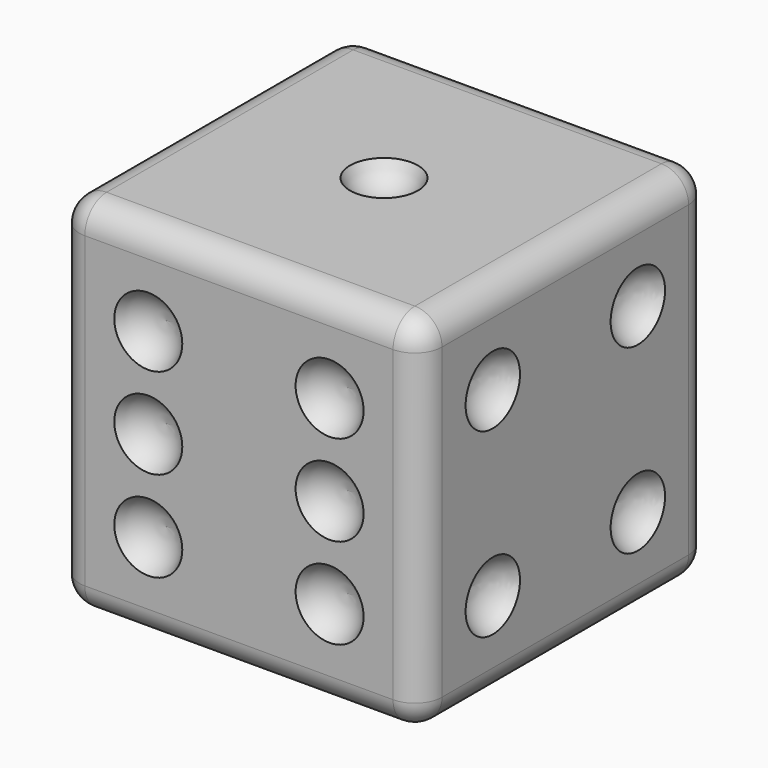
from build123d import *

# Parameters (mm, degrees)
F0_W      = 101.6
F0_H      = 101.6
F0_R      = 9.525
F1_DEPTH  = 101.6
F2_R      = 9.525
F3_DEPTH  = 6.35
F5_R      = 9.525
F6_DEPTH  = 6.35
F8_R      = 9.525
F9_DEPTH  = 6.35
F11_R     = 9.525
F12_DEPTH = 6.35
F14_R     = 9.525
F15_DEPTH = 6.35
F17_R     = 9.525
F18_DEPTH = 6.35
F20_R     = 7.62


# Not quite as in the source:
# - a fillet or chamfer that OpenCascade refuses, or shapes differently, is made with other operations: its cross-section is extruded or revolved along the edge and cut away or added


with BuildPart() as f1:
    # F0 (on Top) → F1 (new body)
    with BuildSketch(Plane.XY):
        with Locations((4.8996444777, 3.5687691152)):
            Rectangle(F0_W, F0_H)
        with Locations((4.8996444777, 3.5687691152)):
            Circle(F0_R, mode=Mode.SUBTRACT)
        with Locations((4.8996444777, 3.5687691152)):
            Circle(F0_R)
    extrude(amount=F1_DEPTH)

    # F2 (on face) → F3 (cut)
    with BuildSketch(Plane.XY.offset(101.6)):
        with Locations((4.8996444777, 3.5687691152)):
            Circle(F2_R)
    extrude(amount=-F3_DEPTH, mode=Mode.SUBTRACT)

    # F4: fillet of radius 10.16 on 1 edges, made by hand

    # F4_s1 → F4_t2 (revolve)
    with BuildSketch(Plane.XZ.offset(-3.5687691152)):
        with BuildLine():
            ThreePointArc((14.4246444777, 101.6), (10.685685062, 96.9857730325), (5.0060723991, 95.25))
            Line((5.0060723991, 95.25), (14.4246444777, 95.25))
            Line((14.4246444777, 95.25), (14.4246444777, 101.6))
        make_face()
    revolve(axis=Axis((4.8996444777, 3.5687691152, 95.25), (0, 0, 1)))

    # F5 (on face) → F6 (cut)
    with BuildSketch(Plane(origin=(-45.9003555223, 0, 0), x_dir=(0, -1, 0), z_dir=(-1, 0, 0))):
        with Locations((-28.9687691152, 25.4)):
            Circle(F5_R)
        with Locations((21.8312308848, 76.2)):
            Circle(F5_R)
    extrude(amount=-F6_DEPTH, mode=Mode.SUBTRACT)

    # F7: fillet of radius 10.16 on 2 edges, made by hand

    # F7_s1 → F7_t2 (revolve)
    with BuildSketch(Plane.XY.offset(25.4)):
        with BuildLine():
            ThreePointArc((-45.9003555223, 19.4437691152), (-41.2861285547, 23.182728531), (-39.5503555223, 28.8623411938))
            Line((-39.5503555223, 28.8623411938), (-39.5503555223, 19.4437691152))
            Line((-39.5503555223, 19.4437691152), (-45.9003555223, 19.4437691152))
        make_face()
    revolve(axis=Axis((-39.5503555223, 28.9687691152, 25.4), (-1, 0, 0)))

    # F7_s3 → F7_t4 (revolve)
    with BuildSketch(Plane.XY.offset(76.2)):
        with BuildLine():
            ThreePointArc((-45.9003555223, -31.3562308848), (-41.2861285547, -27.617271469), (-39.5503555223, -21.9376588062))
            Line((-39.5503555223, -21.9376588062), (-39.5503555223, -31.3562308848))
            Line((-39.5503555223, -31.3562308848), (-45.9003555223, -31.3562308848))
        make_face()
    revolve(axis=Axis((-39.5503555223, -21.8312308848, 76.2), (-1, 0, 0)))

    # F8 (on face) → F9 (cut)
    with BuildSketch(Plane(origin=(0, 0, 0), x_dir=(1, 0, 0), z_dir=(0, 0, -1))):
        with Locations((4.8996444777, -3.5687691152)):
            Circle(F8_R)
        with Locations((30.2996444777, 21.8312308848)):
            Circle(F8_R)
        with Locations((-20.5003555223, -28.9687691152)):
            Circle(F8_R)
    extrude(amount=-F9_DEPTH, mode=Mode.SUBTRACT)

    # F10: fillet of radius 10.16 on 3 edges, made by hand

    # F10_s1 → F10_t2 (revolve)
    with BuildSketch(Plane.XZ.offset(-28.9687691152)):
        with BuildLine():
            ThreePointArc((-10.9753555223, 0), (-14.714314938, 4.6142269675), (-20.3939276009, 6.35))
            Line((-20.3939276009, 6.35), (-10.9753555223, 6.35))
            Line((-10.9753555223, 6.35), (-10.9753555223, 0))
        make_face()
    revolve(axis=Axis((-20.5003555223, 28.9687691152, 6.35), (0, 0, -1)))

    # F10_s3 → F10_t4 (revolve)
    with BuildSketch(Plane.XZ.offset(-3.5687691152)):
        with BuildLine():
            ThreePointArc((14.4246444777, 0), (10.685685062, 4.6142269675), (5.0060723991, 6.35))
            Line((5.0060723991, 6.35), (14.4246444777, 6.35))
            Line((14.4246444777, 6.35), (14.4246444777, 0))
        make_face()
    revolve(axis=Axis((4.8996444777, 3.5687691152, 6.35), (0, 0, -1)))

    # F10_s5 → F10_t6 (revolve)
    with BuildSketch(Plane.XZ.offset(21.8312308848)):
        with BuildLine():
            ThreePointArc((39.8246444777, 0), (36.085685062, 4.6142269675), (30.4060723991, 6.35))
            Line((30.4060723991, 6.35), (39.8246444777, 6.35))
            Line((39.8246444777, 6.35), (39.8246444777, 0))
        make_face()
    revolve(axis=Axis((30.2996444777, -21.8312308848, 6.35), (0, 0, -1)))

    # F11 (on face) → F12 (cut)
    with BuildSketch(Plane.YZ.offset(55.6996444777)):
        with Locations((-21.8312308848, 25.4)):
            Circle(F11_R)
        with Locations((-21.8312308848, 76.2)):
            Circle(F11_R)
        with Locations((28.9687691152, 25.4)):
            Circle(F11_R)
        with Locations((28.9687691152, 76.2)):
            Circle(F11_R)
    extrude(amount=-F12_DEPTH, mode=Mode.SUBTRACT)

    # F13: fillet of radius 10.16 on 4 edges, made by hand

    # F13_s1 → F13_t2 (revolve)
    with BuildSketch(Plane.XY.offset(25.4)):
        with BuildLine():
            ThreePointArc((55.6996444777, 38.4937691152), (51.0854175102, 34.7548096994), (49.3496444777, 29.0751970366))
            Line((49.3496444777, 29.0751970366), (49.3496444777, 38.4937691152))
            Line((49.3496444777, 38.4937691152), (55.6996444777, 38.4937691152))
        make_face()
    revolve(axis=Axis((49.3496444777, 28.9687691152, 25.4), (1, 0, 0)))

    # F13_s3 → F13_t4 (revolve)
    with BuildSketch(Plane.XY.offset(76.2)):
        with BuildLine():
            ThreePointArc((55.6996444777, 38.4937691152), (51.0854175102, 34.7548096994), (49.3496444777, 29.0751970366))
            Line((49.3496444777, 29.0751970366), (49.3496444777, 38.4937691152))
            Line((49.3496444777, 38.4937691152), (55.6996444777, 38.4937691152))
        make_face()
    revolve(axis=Axis((49.3496444777, 28.9687691152, 76.2), (1, 0, 0)))

    # F13_s5 → F13_t6 (revolve)
    with BuildSketch(Plane.XY.offset(76.2)):
        with BuildLine():
            ThreePointArc((55.6996444777, -12.3062308848), (51.0854175102, -16.0451903006), (49.3496444777, -21.7248029634))
            Line((49.3496444777, -21.7248029634), (49.3496444777, -12.3062308848))
            Line((49.3496444777, -12.3062308848), (55.6996444777, -12.3062308848))
        make_face()
    revolve(axis=Axis((49.3496444777, -21.8312308848, 76.2), (1, 0, 0)))

    # F13_s7 → F13_t8 (revolve)
    with BuildSketch(Plane.XY.offset(25.4)):
        with BuildLine():
            ThreePointArc((55.6996444777, -12.3062308848), (51.0854175102, -16.0451903006), (49.3496444777, -21.7248029634))
            Line((49.3496444777, -21.7248029634), (49.3496444777, -12.3062308848))
            Line((49.3496444777, -12.3062308848), (55.6996444777, -12.3062308848))
        make_face()
    revolve(axis=Axis((49.3496444777, -21.8312308848, 25.4), (1, 0, 0)))

    # F14 (on face) → F15 (cut)
    with BuildSketch(Plane(origin=(0, 54.3687691152, 0), x_dir=(-1, 0, 0), z_dir=(0, 1, 0))):
        with Locations((-4.8996444777, 50.8)):
            Circle(F14_R)
        with Locations((-30.2996444777, 25.4)):
            Circle(F14_R)
        with Locations((20.5003555223, 76.2)):
            Circle(F14_R)
        with Locations((-30.2996444777, 76.2)):
            Circle(F14_R)
        with Locations((20.5003555223, 25.4)):
            Circle(F14_R)
    extrude(amount=-F15_DEPTH, mode=Mode.SUBTRACT)

    # F16: fillet of radius 10.16 on 5 edges, made by hand

    # F16_s1 → F16_t2 (revolve)
    with BuildSketch(Plane.XY.offset(25.4)):
        with BuildLine():
            ThreePointArc((-30.0253555223, 54.3687691152), (-26.2863961065, 49.7545421477), (-20.6067834436, 48.0187691152))
            Line((-20.6067834436, 48.0187691152), (-30.0253555223, 48.0187691152))
            Line((-30.0253555223, 48.0187691152), (-30.0253555223, 54.3687691152))
        make_face()
    revolve(axis=Axis((-20.5003555223, 48.0187691152, 25.4), (0, 1, 0)))

    # F16_s3 → F16_t4 (revolve)
    with BuildSketch(Plane.XY.offset(50.8)):
        with BuildLine():
            ThreePointArc((-4.6253555223, 54.3687691152), (-0.8863961065, 49.7545421477), (4.7932165564, 48.0187691152))
            Line((4.7932165564, 48.0187691152), (-4.6253555223, 48.0187691152))
            Line((-4.6253555223, 48.0187691152), (-4.6253555223, 54.3687691152))
        make_face()
    revolve(axis=Axis((4.8996444777, 48.0187691152, 50.8), (0, 1, 0)))

    # F16_s5 → F16_t6 (revolve)
    with BuildSketch(Plane.XY.offset(76.2)):
        with BuildLine():
            ThreePointArc((-30.0253555223, 54.3687691152), (-26.2863961065, 49.7545421477), (-20.6067834436, 48.0187691152))
            Line((-20.6067834436, 48.0187691152), (-30.0253555223, 48.0187691152))
            Line((-30.0253555223, 48.0187691152), (-30.0253555223, 54.3687691152))
        make_face()
    revolve(axis=Axis((-20.5003555223, 48.0187691152, 76.2), (0, 1, 0)))

    # F16_s7 → F16_t8 (revolve)
    with BuildSketch(Plane.XY.offset(76.2)):
        with BuildLine():
            ThreePointArc((20.7746444777, 54.3687691152), (24.5136038935, 49.7545421477), (30.1932165564, 48.0187691152))
            Line((30.1932165564, 48.0187691152), (20.7746444777, 48.0187691152))
            Line((20.7746444777, 48.0187691152), (20.7746444777, 54.3687691152))
        make_face()
    revolve(axis=Axis((30.2996444777, 48.0187691152, 76.2), (0, 1, 0)))

    # F16_s9 → F16_t10 (revolve)
    with BuildSketch(Plane.XY.offset(25.4)):
        with BuildLine():
            ThreePointArc((20.7746444777, 54.3687691152), (24.5136038935, 49.7545421477), (30.1932165564, 48.0187691152))
            Line((30.1932165564, 48.0187691152), (20.7746444777, 48.0187691152))
            Line((20.7746444777, 48.0187691152), (20.7746444777, 54.3687691152))
        make_face()
    revolve(axis=Axis((30.2996444777, 48.0187691152, 25.4), (0, 1, 0)))

    # F17 (on face) → F18 (cut)
    with BuildSketch(Plane.XZ.offset(47.2312308848)):
        with Locations((30.2996444777, 25.4)):
            Circle(F17_R)
        with Locations((30.2996444777, 50.8)):
            Circle(F17_R)
        with Locations((30.2996444777, 76.2)):
            Circle(F17_R)
        with Locations((-20.5003555223, 25.4)):
            Circle(F17_R)
        with Locations((-20.5003555223, 50.8)):
            Circle(F17_R)
        with Locations((-20.5003555223, 76.2)):
            Circle(F17_R)
    extrude(amount=-F18_DEPTH, mode=Mode.SUBTRACT)

    # F19: fillet of radius 10.16 on 6 edges, made by hand

    # F19_s1 → F19_t2 (revolve)
    with BuildSketch(Plane.XY.offset(25.4)):
        with BuildLine():
            ThreePointArc((39.8246444777, -47.2312308848), (36.085685062, -42.6170039173), (30.4060723991, -40.8812308848))
            Line((30.4060723991, -40.8812308848), (39.8246444777, -40.8812308848))
            Line((39.8246444777, -40.8812308848), (39.8246444777, -47.2312308848))
        make_face()
    revolve(axis=Axis((30.2996444777, -40.8812308848, 25.4), (0, -1, 0)))

    # F19_s3 → F19_t4 (revolve)
    with BuildSketch(Plane.XY.offset(50.8)):
        with BuildLine():
            ThreePointArc((39.8246444777, -47.2312308848), (36.085685062, -42.6170039173), (30.4060723991, -40.8812308848))
            Line((30.4060723991, -40.8812308848), (39.8246444777, -40.8812308848))
            Line((39.8246444777, -40.8812308848), (39.8246444777, -47.2312308848))
        make_face()
    revolve(axis=Axis((30.2996444777, -40.8812308848, 50.8), (0, -1, 0)))

    # F19_s5 → F19_t6 (revolve)
    with BuildSketch(Plane.XY.offset(76.2)):
        with BuildLine():
            ThreePointArc((39.8246444777, -47.2312308848), (36.085685062, -42.6170039173), (30.4060723991, -40.8812308848))
            Line((30.4060723991, -40.8812308848), (39.8246444777, -40.8812308848))
            Line((39.8246444777, -40.8812308848), (39.8246444777, -47.2312308848))
        make_face()
    revolve(axis=Axis((30.2996444777, -40.8812308848, 76.2), (0, -1, 0)))

    # F19_s7 → F19_t8 (revolve)
    with BuildSketch(Plane.XY.offset(76.2)):
        with BuildLine():
            ThreePointArc((-10.9753555223, -47.2312308848), (-14.714314938, -42.6170039173), (-20.3939276009, -40.8812308848))
            Line((-20.3939276009, -40.8812308848), (-10.9753555223, -40.8812308848))
            Line((-10.9753555223, -40.8812308848), (-10.9753555223, -47.2312308848))
        make_face()
    revolve(axis=Axis((-20.5003555223, -40.8812308848, 76.2), (0, -1, 0)))

    # F19_s9 → F19_t10 (revolve)
    with BuildSketch(Plane.XY.offset(50.8)):
        with BuildLine():
            ThreePointArc((-10.9753555223, -47.2312308848), (-14.714314938, -42.6170039173), (-20.3939276009, -40.8812308848))
            Line((-20.3939276009, -40.8812308848), (-10.9753555223, -40.8812308848))
            Line((-10.9753555223, -40.8812308848), (-10.9753555223, -47.2312308848))
        make_face()
    revolve(axis=Axis((-20.5003555223, -40.8812308848, 50.8), (0, -1, 0)))

    # F19_s11 → F19_t12 (revolve)
    with BuildSketch(Plane.XY.offset(25.4)):
        with BuildLine():
            ThreePointArc((-10.9753555223, -47.2312308848), (-14.714314938, -42.6170039173), (-20.3939276009, -40.8812308848))
            Line((-20.3939276009, -40.8812308848), (-10.9753555223, -40.8812308848))
            Line((-10.9753555223, -40.8812308848), (-10.9753555223, -47.2312308848))
        make_face()
    revolve(axis=Axis((-20.5003555223, -40.8812308848, 25.4), (0, -1, 0)))

    # F20
    f20_edges = [f1.edges().sort_by_distance(p)[0] for p in [
        (55.699644, 3.568769, 101.6),
        (4.899644, 54.368769, 101.6),
        (55.699644, 54.368769, 50.8),
        (4.899644, -47.231231, 101.6),
        (-45.900356, 3.568769, 101.6),
        (55.699644, 3.568769, 0),
        (4.899644, 54.368769, 0),
        (4.899644, -47.231231, 0),
        (-45.900356, 3.568769, 0),
        (55.699644, -47.231231, 50.8),
        (-45.900356, -47.231231, 50.8),
        (-45.900356, 54.368769, 50.8),
    ]]
    fillet(f20_edges, radius=F20_R)


solid = f1.part
